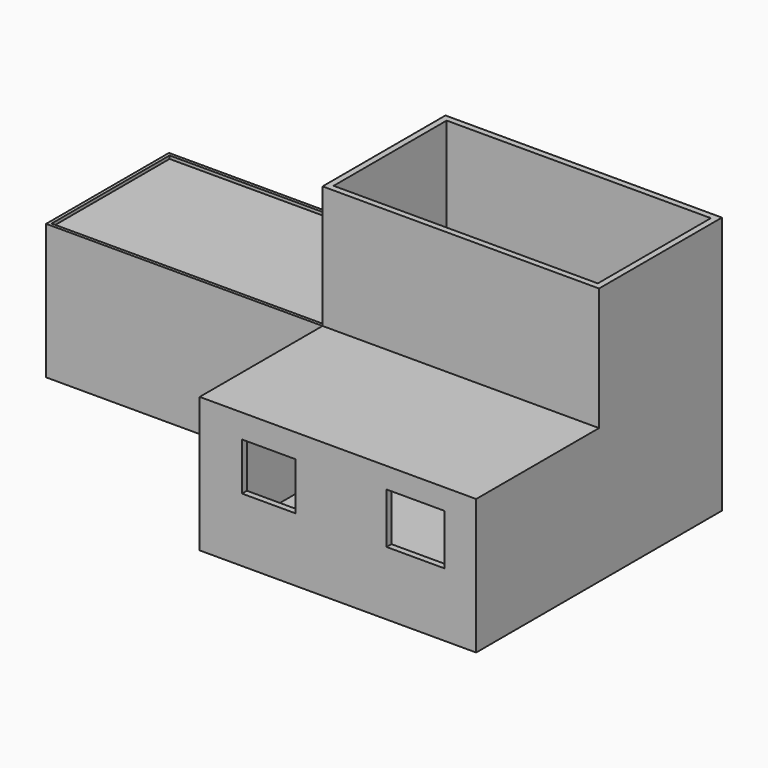
from build123d import *

# Parameters (mm, degrees)
F0_W         = 4500
F0_H         = 2500
F1_DEPTH     = 4200
F2_DEPTH     = 2200
F3_DEPTH     = 2200
F4_T         = -100
F5_T         = 50
F5_T3_DEPTH  = 2300
F5_T5_DEPTH  = 4600
F5_T7_DEPTH  = 2200
F5_T9_DEPTH  = 4200
F5_T11_DEPTH = 8900
F5_T13_DEPTH = 2100
F5_T15_DEPTH = 4600
F5_T17_DEPTH = 4900
F5_T19_DEPTH = 4400
F5_T21_DEPTH = 2600
F5_T23_DEPTH = 2400
F6_W         = 868.8530921936
F6_H         = 775.7483720779
F6_W_2       = 941.2586688995
F6_H_2       = 824.3043422699
F7_DEPTH     = 100


# Not quite as in the source:
# - a shell that OpenCascade refuses in one call is made with other operations: the cavity is built on its own and cut out


with BuildPart() as f1:
    # F0 (on Top) → F1 (new body)
    with BuildSketch(Plane.XY):
        with Locations((2250, 1250)):
            Rectangle(F0_W, F0_H)
    extrude(amount=F1_DEPTH)

    # F0 (on Top) → F2 (join)
    with BuildSketch(Plane.XY):
        with Locations((2250, -1250)):
            Rectangle(F0_W, F0_H)
    extrude(amount=F2_DEPTH)

    # F0 (on Top) → F3 (join)
    with BuildSketch(Plane.XY):
        with Locations((-2250, 1250)):
            Rectangle(F0_W, F0_H)
    extrude(amount=F3_DEPTH)

    # F4
    f4_openings = [f1.faces().sort_by_distance(p)[0] for p in [
        (2250, 1250, 4200),
    ]]
    offset(amount=F4_T, openings=f4_openings, kind=Kind.INTERSECTION)

    # F5: shell of thickness 50, made by hand


with BuildPart() as f5_core1:
    # F5_t2: copy of F1
    add(f1.part)

    # the walls: a layer under each face that stays
    f5_faces = [f5_core1.faces().sort_by_distance(p)[0] for p in [
        (0, 1250, 3200),
        (0, 2500, 2100),
        (-3000, 1666.6666666667, 0),
        (-2250, 0, 1100),
        (2250, -2500, 1100),
        (2250, -1250, 2200),
        (0, -1250, 1100),
        (-4500, 1250, 1100),
        (4500, 0, 2100),
        (2250, 0, 3200),
        (150, 83.3333333333, 4200),
        (100, 1250, 3150),
        (2933.3333333333, 2400, 3516.6666666667),
        (-2933.3333333333, 1600, 100),
        (-2150, 100, 1100),
        (2250, -2400, 1100),
        (2250, -1150, 2100),
        (100, -1150, 1100),
        (-4400, 1250, 1100),
        (4400, -1600, 783.3333333333),
        (2250, 100, 3150),
        (-2150, 1250, 2100),
    ]]
    thicken(f5_faces, amount=-F5_T, mode=Mode.SUBTRACT)

    # F5_s4 → F5_t3 (cut)
    with BuildSketch(Plane.XY.offset(-50)):
        Polygon((-0.5, -0.5), (0, 50), (50, 50), (50, 0), align=None)
    extrude(amount=F5_T3_DEPTH, mode=Mode.SUBTRACT)

    # F5_s6 → F5_t5 (cut)
    with BuildSketch(Plane.YZ.offset(-50)):
        Polygon((-0.5, 2200.5), (0, 2150), (50, 2150), (50, 2200), align=None)
    extrude(amount=F5_T5_DEPTH, mode=Mode.SUBTRACT)

    # F5_s8 → F5_t7 (cut)
    with BuildSketch(Plane.XY.offset(2050)):
        Polygon((100.5, 100.5), (50, 100), (50, 50), (100, 50), align=None)
        Polygon((100.5, 2399.5), (50, 2400), (50, 2450), (100, 2450), align=None)
        Polygon((4399.5, 100.5), (4450, 100), (4450, 50), (4400, 50), align=None)
    extrude(amount=F5_T7_DEPTH, mode=Mode.SUBTRACT)

    # F5_s10 → F5_t9 (cut)
    with BuildSketch(Plane.XY.offset(50)):
        Polygon((4399.5, 2399.5), (4400, 2450), (4450, 2450), (4450, 2400), align=None)
    extrude(amount=F5_T9_DEPTH, mode=Mode.SUBTRACT)

    # F5_s12 → F5_t11 (cut)
    with BuildSketch(Plane.YZ.offset(-4450)):
        Polygon((2399.5, 100.5), (2450, 100), (2450, 50), (2400, 50), align=None)
    extrude(amount=F5_T11_DEPTH, mode=Mode.SUBTRACT)

    # F5_s14 → F5_t13 (cut)
    with BuildSketch(Plane.XY.offset(50)):
        Polygon((-4399.5, 2399.5), (-4400, 2450), (-4450, 2450), (-4450, 2400), align=None)
        Polygon((-4399.5, 100.5), (-4400, 50), (-4450, 50), (-4450, 100), align=None)
        Polygon((4399.5, -2399.5), (4400, -2450), (4450, -2450), (4450, -2400), align=None)
        Polygon((100.5, -2399.5), (100, -2450), (50, -2450), (50, -2400), align=None)
    extrude(amount=F5_T13_DEPTH, mode=Mode.SUBTRACT)

    # F5_s16 → F5_t15 (cut)
    with BuildSketch(Plane.YZ.offset(-4450)):
        Polygon((2399.5, 2099.5), (2450, 2100), (2450, 2150), (2400, 2150), align=None)
        Polygon((100.5, 100.5), (100, 50), (50, 50), (50, 100), align=None)
        Polygon((100.5, 2099.5), (50, 2100), (50, 2150), (100, 2150), align=None)
    extrude(amount=F5_T15_DEPTH, mode=Mode.SUBTRACT)

    # F5_s18 → F5_t17 (cut)
    with BuildSketch(Plane.XZ.offset(-2450)):
        Polygon((4399.5, 100.5), (4400, 50), (4450, 50), (4450, 100), align=None)
    extrude(amount=F5_T17_DEPTH, mode=Mode.SUBTRACT)

    # F5_s20 → F5_t19 (cut)
    with BuildSketch(Plane.YZ.offset(50)):
        Polygon((-2399.5, 100.5), (-2400, 50), (-2450, 50), (-2450, 100), align=None)
        Polygon((-2399.5, 2099.5), (-2450, 2100), (-2450, 2150), (-2400, 2150), align=None)
    extrude(amount=F5_T19_DEPTH, mode=Mode.SUBTRACT)

    # F5_s22 → F5_t21 (cut)
    with BuildSketch(Plane.XZ.offset(-150)):
        Polygon((100.5, 100.5), (100, 50), (50, 50), (50, 100), align=None)
        Polygon((100.5, 2099.5), (100, 2150), (50, 2150), (50, 2100), align=None)
        Polygon((4399.5, 2099.5), (4400, 2150), (4450, 2150), (4450, 2100), align=None)
    extrude(amount=F5_T21_DEPTH, mode=Mode.SUBTRACT)

    # F5_s24 → F5_t23 (cut)
    with BuildSketch(Plane.XZ.offset(-2450)):
        Polygon((-4399.5, 100.5), (-4400, 50), (-4450, 50), (-4450, 100), align=None)
        Polygon((-4399.5, 2099.5), (-4450, 2100), (-4450, 2150), (-4400, 2150), align=None)
    extrude(amount=F5_T23_DEPTH, mode=Mode.SUBTRACT)


with BuildPart() as f1_1:
    add(f1.part)

    # what is left inside the walls is the cavity
    f5_cavity = [f5_core1.part.solids().sort_by_distance(p)[0] for p in [
        (-2200, 850, 2199.5),
    ]]
    add(f5_cavity, mode=Mode.SUBTRACT)

    # F6 (on face) → F7 (cut, through all)
    with BuildSketch(Plane.XZ.offset(2500)):
        with Locations((1123.2978105545, 1426.2890219688)):
            Rectangle(F6_W, F6_H)
        with Locations((3512.6439332962, 1450.5670070648)):
            Rectangle(F6_W_2, F6_H_2)
    extrude(amount=-F7_DEPTH, mode=Mode.SUBTRACT)


solid = f1_1.part
